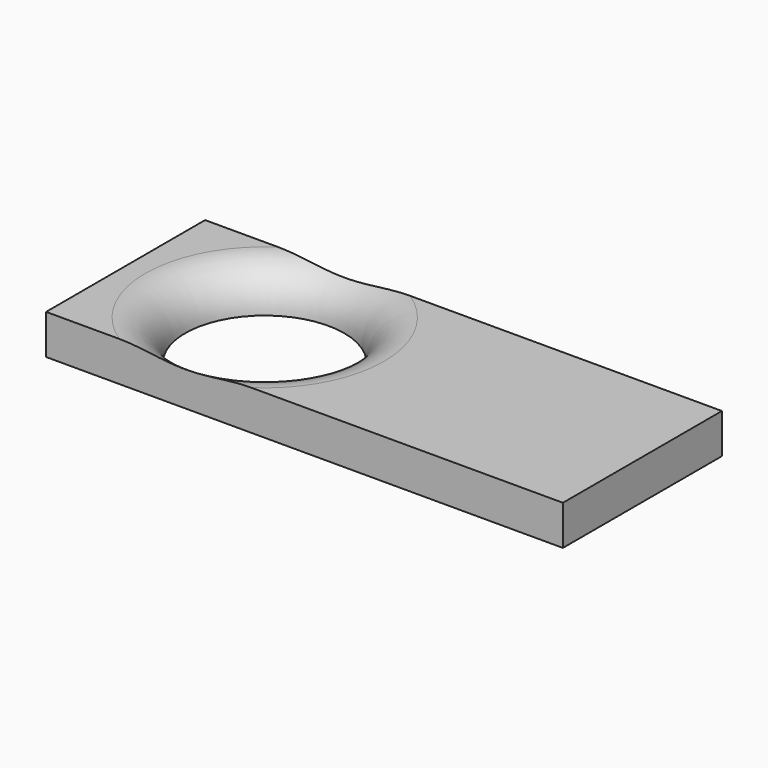
from build123d import *

# Parameters (mm, degrees)
F0_W     = 330.2
F0_H     = 127
F0_R     = 50.8
F1_DEPTH = 25.4


# Not quite as in the source:
# - a fillet or chamfer that OpenCascade refuses, or shapes differently, is made with other operations: its cross-section is extruded or revolved along the edge and cut away or added


with BuildPart() as f1:
    # F0 (on Top) → F1 (new body)
    with BuildSketch(Plane.XY):
        Rectangle(F0_W, F0_H)
        with Locations((-76.2, 0)):
            Circle(F0_R, mode=Mode.SUBTRACT)
    extrude(amount=F1_DEPTH)

    # F2: fillet of radius 25.4 on 1 edges, made by hand

    # F2_s1 → F2_t2 (revolve, cut)
    with BuildSketch(Plane.XZ):
        with BuildLine():
            ThreePointArc((-25.4, 0), (-17.9605122421, 17.9605122421), (0, 25.4))
            Line((0, 25.4), (-25.4, 25.4))
            Line((-25.4, 25.4), (-25.4, 0))
        make_face()
    revolve(axis=Axis((-76.2, 0, 25.4), (0, 0, 1)), mode=Mode.SUBTRACT)


solid = f1.part
